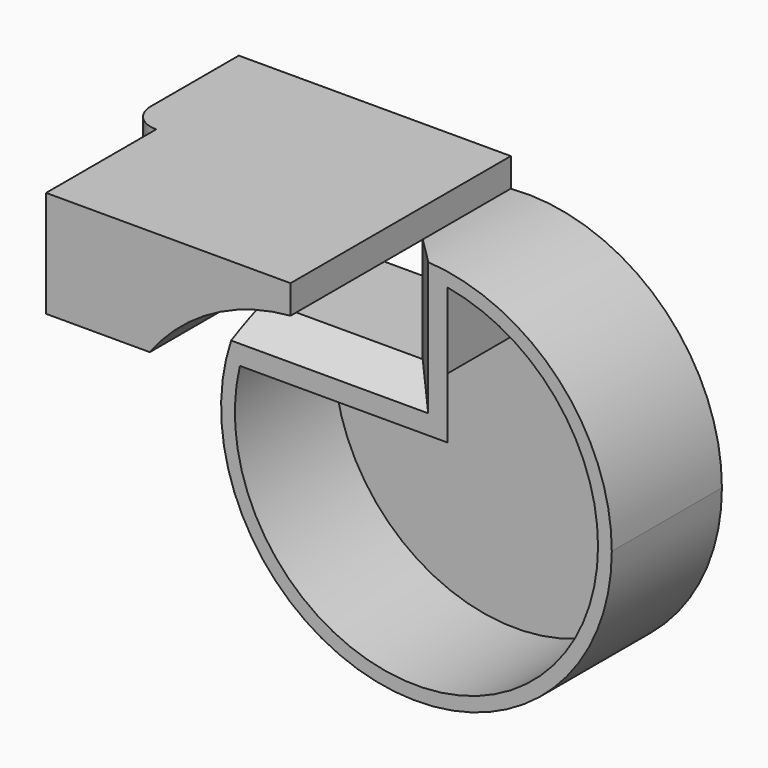
from build123d import *

# Parameters (mm, degrees)
F1_DEPTH = 25.4
F2_R     = 5.08
F3_SIZE  = 5.08
F4_T     = -2.54
F5_DEPTH = 25.4


with BuildPart() as f1:
    # F0 (on Front) → F1 (new body)
    with BuildSketch(Plane.XZ):
        with BuildLine():
            ThreePointArc((-32.0517227431, 16.4869092405), (-20.0009755061, 29.9848642803), (-2.9094549827, 35.925842771))
            Line((-2.9094549827, 35.925842771), (-2.9094549827, 41.2172712386))
            Line((-2.9094549827, 41.2172712386), (-53.0975461006, 41.2172712386))
            Line((-53.0975461006, 41.2172712386), (-53.0975461006, 16.4869092405))
            Line((-53.0975461006, 16.4869092405), (-32.0517227431, 16.4869092405))
        make_face()
    extrude(amount=F1_DEPTH)

    # F2
    f2_edges = [f1.edges().sort_by_distance(p)[0] for p in [
        (-53.097546, -25.4, 28.85209),
        (-42.574634, -25.4, 16.486909),
    ]]
    fillet(f2_edges, radius=F2_R)

    # F5 (add): a face of the model
    f5_faces = [f1.faces().sort_by_distance(p)[0] for p in [
        (-30.4342357223, -25.4, 33.0216663243),
    ]]
    extrude(f5_faces, amount=F5_DEPTH)


with BuildPart() as f1b:
    # F0 (on Front) → F1, piece 2 (new body)
    with BuildSketch(Plane.XZ):
        with BuildLine():
            ThreePointArc((-32.0517227431, 16.4869092405), (-8.4816294649, -35.0313155437), (36.0434613641, 0))
            ThreePointArc((36.0434613641, 0), (24.4362873494, 26.4952631178), (-2.9094549827, 35.925842771))
            Line((-2.9094549827, 35.925842771), (-2.9094549827, 16.4869092405))
            Line((-2.9094549827, 16.4869092405), (-32.0517227431, 16.4869092405))
        make_face()
    extrude(amount=F1_DEPTH)

    # F3
    f3_edges = [f1b.edges().sort_by_distance(p)[0] for p in [
        (-17.480589, -25.4, 16.486909),
        (-2.909455, -25.4, 26.206376),
    ]]
    chamfer(f3_edges, length=F3_SIZE)

    # F4
    f4_openings = [f1b.faces().sort_by_distance(p)[0] for p in [
        (2.458641, -25.4, -4.276447),
    ]]
    offset(amount=F4_T, openings=f4_openings, kind=Kind.INTERSECTION)


solid = Compound([f1.part, f1b.part])
